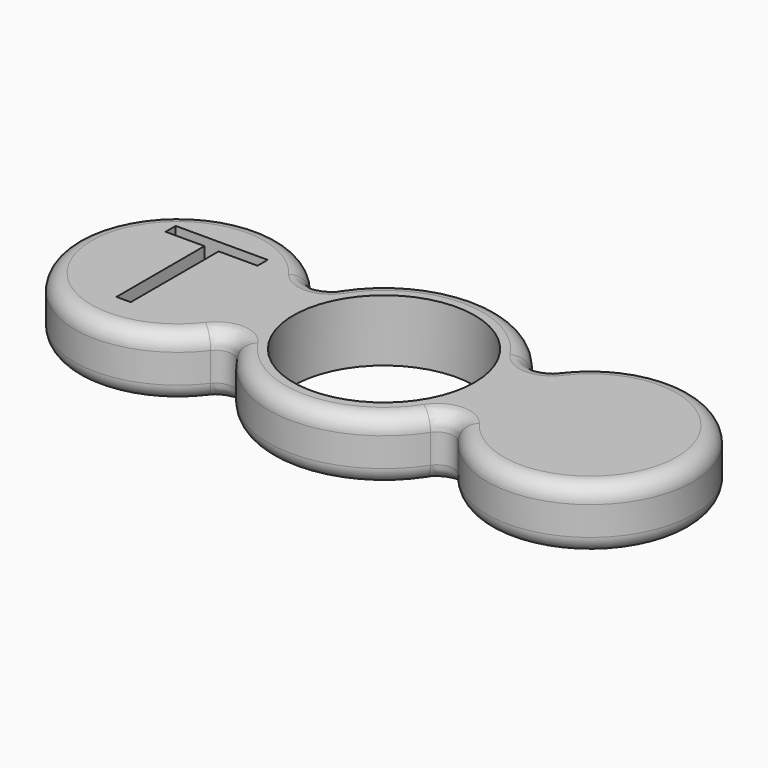
from build123d import *

# Parameters (mm, degrees)
F0_R         = 11
F1_DEPTH     = 7.5
F2_R         = 2
F3_R         = 2
F4_TEXT_SIZE = 20.8333333333
F5_DEPTH     = 25


# Not quite as in the source:
# - Text() gives the source's letters only with a copy of the font that has no kerning and outlines rounded to 1/6400 em; it was checked with that copy


with BuildPart() as f1:
    # F0 (on Top) → F1 (new body)
    with BuildSketch(Plane.XY):
        with BuildLine():
            ThreePointArc((-13.295, 4.3866815476), (-37.5, 0), (-13.295, -4.3866815476))
            ThreePointArc((-13.295, -4.3866815476), (0, -14), (13.295, -4.3866815476))
            ThreePointArc((13.295, -4.3866815476), (37.5, 0), (13.295, 4.3866815476))
            ThreePointArc((13.295, 4.3866815476), (0, 14), (-13.295, 4.3866815476))
        make_face()
        Circle(F0_R, mode=Mode.SUBTRACT)
    extrude(amount=F1_DEPTH)

    # F2
    f2_edges = [f1.edges().sort_by_distance(p)[0] for p in [
        (-13.295, -4.386682, 3.75),
        (13.295, -4.386682, 3.75),
        (13.295, 4.386682, 3.75),
        (-13.295, 4.386682, 3.75),
    ]]
    fillet(f2_edges, radius=F2_R)

    # F3
    f3_edges = [f1.edges().sort_by_distance(p)[0] for p in [
        (-37.5, 0, 7.5),
        (-37.5, 0, 0),
    ]]
    fillet(f3_edges, radius=F3_R)

    # F4 (on face) → F5 (cut)
    with BuildSketch(Plane.XY.offset(7.5)):
        with Locations((-31.3411458333, -7.5)):
            Text('T', F4_TEXT_SIZE, font='Open Sans', text_align=(TextAlign.LEFT, TextAlign.BOTTOM))
    extrude(amount=-F5_DEPTH, mode=Mode.SUBTRACT)


solid = f1.part
